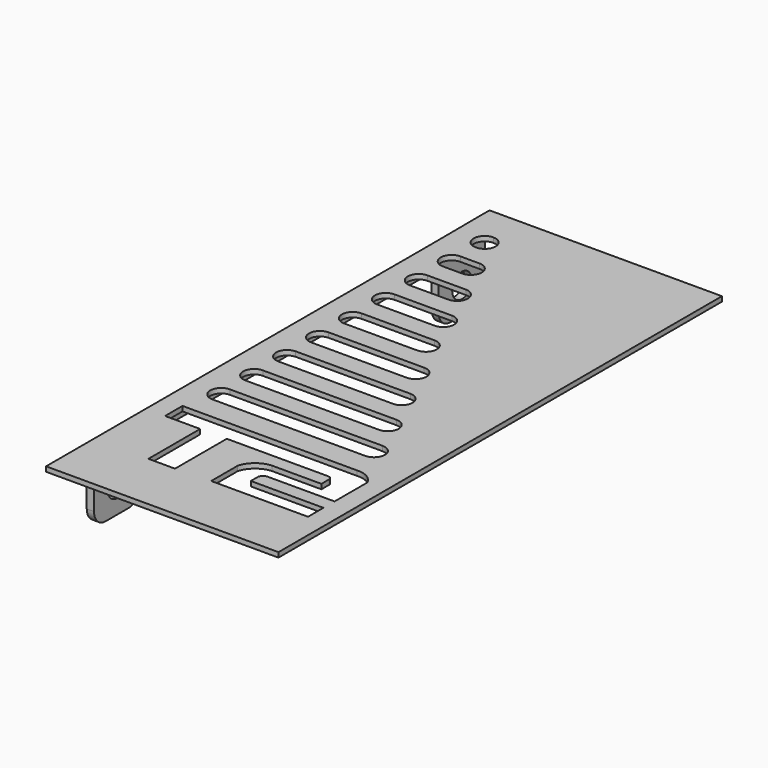
from build123d import *

# Parameters (mm, degrees)
F1_DEPTH = 1
F2_DEPTH = 15
F4_D     = 5
F5_R     = 3
F6_DEPTH = 4


# Not quite as in the source:
# - a feature names something its author has since deleted; it is built from what else it names


with BuildPart() as f1:
    # F0 (on Top) → F1 (new body)
    with BuildSketch(Plane.XY):
        Polygon((24, 57.25), (-24, 57.25), (-24.0091441598, 54.25), (-22.5091511277, 54.2454279414), (-22.5091511277, 42.2454279414), (-22.5, -34.75), (-22.5, -46.75), (-24, -46.75), (-24, -57.25), (24, -57.25), align=None)
        with BuildLine():
            Line((13.9209458456, -22.2416133583), (-17.6390541544, -22.2416133583))
            ThreePointArc((-17.6390541544, -22.2416133583), (-19.8890541544, -19.9916133583), (-17.6390541544, -17.7416133583))
            Line((-17.6390541544, -17.7416133583), (13.9209458456, -17.7416133583))
            ThreePointArc((13.9209458456, -17.7416133583), (16.1709458456, -19.9916133583), (13.9209458456, -22.2416133583))
        make_face(mode=Mode.SUBTRACT)
        with BuildLine():
            Line((9.9809458456, -13.7416133583), (-17.6390541544, -13.7416133583))
            ThreePointArc((-17.6390541544, -13.7416133583), (-19.8890541544, -11.4916133583), (-17.6390541544, -9.2416133583))
            Line((-17.6390541544, -9.2416133583), (9.9809458456, -9.2416133583))
            ThreePointArc((9.9809458456, -9.2416133583), (12.2309458456, -11.4916133583), (9.9809458456, -13.7416133583))
        make_face(mode=Mode.SUBTRACT)
        with BuildLine():
            Line((6.0409458456, -5.2416133583), (-17.6390541544, -5.2416133583))
            ThreePointArc((-17.6390541544, -5.2416133583), (-19.8890541544, -2.9916133583), (-17.6390541544, -0.7416133583))
            Line((-17.6390541544, -0.7416133583), (6.0409458456, -0.7416133583))
            ThreePointArc((6.0409458456, -0.7416133583), (8.2909458456, -2.9916133583), (6.0409458456, -5.2416133583))
        make_face(mode=Mode.SUBTRACT)
        with BuildLine():
            Line((-19.9999999992, -31.5317022603), (-19.9999999992, -27.0317022603))
            Line((-19.9999999992, -27.0317022603), (16.0951670268, -27.0317022603))
            ThreePointArc((16.0951670268, -27.0317022603), (18.3824934665, -27.555243649), (19.9999999704, -29.25513498))
            Line((19.9999999704, -29.25513498), (19.991580365, -37.75513498))
            Line((19.991580365, -37.75513498), (6.1573753969, -37.7551350426))
            ThreePointArc((6.1573753969, -37.7551350426), (5.4441089744, -38.037790108), (4.9890264818, -38.6554816172))
            Line((4.9890264818, -38.6554816172), (4.9890264818, -40.6197120801))
            Line((4.9890264818, -40.6197120801), (19.9890264818, -40.6197120801))
            Line((19.9890264818, -40.6197120801), (20, -44.6197120801))
            Line((20, -44.6197120801), (0, -44.6197120801))
            Line((0, -44.6197120801), (0, -37.7900532508))
            ThreePointArc((0, -37.7900532508), (1.5958871284, -35.3350022858), (4.3312619815, -34.2900834468))
            Line((4.3312619815, -34.2900834468), (14.5000001306, -34.2900834468))
            Line((14.5000001306, -34.2900834468), (14.5000000048, -32.3122422563))
            ThreePointArc((14.5000000048, -32.3122422563), (14.2713851276, -31.7603171319), (13.7194600008, -31.5317022603))
            Line((13.7194600008, -31.5317022603), (-7.2499999992, -31.5317022603))
            Line((-7.2499999992, -31.5317022603), (-7.2499999992, -44.8960133593))
            Line((-7.2499999992, -44.8960133593), (-12.7499999992, -44.8960133593))
            Line((-12.7499999992, -44.8960133593), (-12.7499999992, -31.5317022603))
            Line((-12.7499999992, -31.5317022603), (-19.9999999992, -31.5317022603))
        make_face(mode=Mode.SUBTRACT)
        with BuildLine():
            Line((2.1009458456, 3.2583866417), (-17.6390541544, 3.2583866417))
            ThreePointArc((-17.6390541544, 3.2583866417), (-19.8890541544, 5.5083866417), (-17.6390541544, 7.7583866417))
            Line((-17.6390541544, 7.7583866417), (2.1009458456, 7.7583866417))
            ThreePointArc((2.1009458456, 7.7583866417), (4.3509458456, 5.5083866417), (2.1009458456, 3.2583866417))
        make_face(mode=Mode.SUBTRACT)
        with BuildLine():
            Line((-2.5590541544, 11.7583866417), (-17.6390541544, 11.7583866417))
            ThreePointArc((-17.6390541544, 11.7583866417), (-19.8890541544, 14.0083866417), (-17.6390541544, 16.2583866417))
            Line((-17.6390541544, 16.2583866417), (-2.5590541544, 16.2583866417))
            ThreePointArc((-2.5590541544, 16.2583866417), (-0.3090541544, 14.0083866417), (-2.5590541544, 11.7583866417))
        make_face(mode=Mode.SUBTRACT)
        with BuildLine():
            Line((-5.7790541544, 20.2583866417), (-17.6390541544, 20.2583866417))
            ThreePointArc((-17.6390541544, 20.2583866417), (-19.8890541544, 22.5083866417), (-17.6390541544, 24.7583866417))
            Line((-17.6390541544, 24.7583866417), (-5.7790541544, 24.7583866417))
            ThreePointArc((-5.7790541544, 24.7583866417), (-3.5290541544, 22.5083866417), (-5.7790541544, 20.2583866417))
        make_face(mode=Mode.SUBTRACT)
        with BuildLine():
            Line((-9.7190541544, 28.7583866417), (-17.6390541544, 28.7583866417))
            ThreePointArc((-17.6390541544, 28.7583866417), (-19.8890541544, 31.0083866417), (-17.6390541544, 33.2583866417))
            Line((-17.6390541544, 33.2583866417), (-9.7190541544, 33.2583866417))
            ThreePointArc((-9.7190541544, 33.2583866417), (-7.4690541544, 31.0083866417), (-9.7190541544, 28.7583866417))
        make_face(mode=Mode.SUBTRACT)
        with BuildLine():
            Line((-13.6590541544, 37.2583866417), (-17.6390541544, 37.2583866417))
            ThreePointArc((-17.6390541544, 37.2583866417), (-19.8890541544, 39.5083866417), (-17.6390541544, 41.7583866417))
            Line((-17.6390541544, 41.7583866417), (-13.6590541544, 41.7583866417))
            ThreePointArc((-13.6590541544, 41.7583866417), (-11.4090541544, 39.5083866417), (-13.6590541544, 37.2583866417))
        make_face(mode=Mode.SUBTRACT)
        with BuildLine():
            Line((-17.5990541544, 45.7583866417), (-17.6390541544, 45.7583866417))
            ThreePointArc((-17.6390541544, 45.7583866417), (-19.8890541544, 48.0083866417), (-17.6390541544, 50.2583866417))
            Line((-17.6390541544, 50.2583866417), (-17.5990541544, 50.2583866417))
            ThreePointArc((-17.5990541544, 50.2583866417), (-15.3490541544, 48.0083866417), (-17.5990541544, 45.7583866417))
        make_face(mode=Mode.SUBTRACT)
    extrude(amount=-F1_DEPTH)

    # F0 (on Top) → F2 (join)
    with BuildSketch(Plane.XY):
        Polygon((-22.5091511277, 54.2454279414), (-24.0091441598, 54.25), (-23.9357289877, 42.2454279414), (-22.5091511277, 42.2454279414), align=None)
        Polygon((-22.5, -34.75), (-23.997312058, -34.750000301), (-24, -46.75), (-22.5, -46.75), align=None)
    extrude(amount=-F2_DEPTH)

    # F4 (through all)
    with Locations(Plane.YZ):
        with Locations((-40.75, -9.5), (48.25, -9.5)):
            Hole(F4_D / 2)

    # F5
    f5_edges = [f1.edges().sort_by_distance(p)[0] for p in [
        (-23.22244, 42.245428, -15),
        (-23.259148, 54.247714, -15),
        (-23.248656, -34.75, -15),
        (-23.25, -46.75, -15),
    ]]
    fillet(f5_edges, radius=F5_R)

    # F0 (on Top) → F6 (join)
    with BuildSketch(Plane.XY):
        Polygon((-22.5091511277, 42.2454279414), (-23.9357289877, 42.2454279414), (-23.997312058, -34.750000301), (-22.5, -34.75), align=None)
    extrude(amount=-F6_DEPTH)


solid = f1.part
